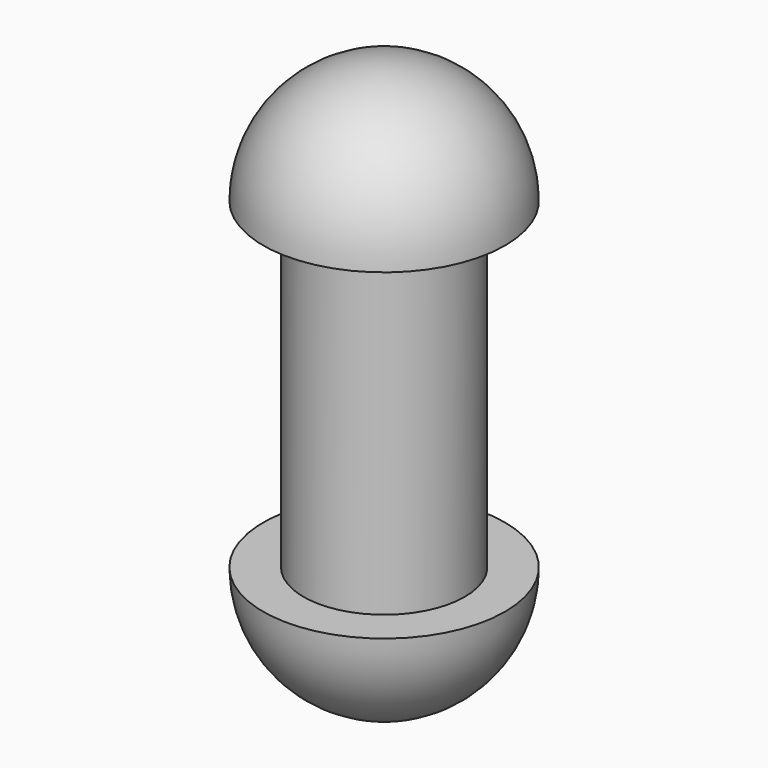
from build123d import *

# Parameters (mm, degrees)
F0_R     = 1
F1_DEPTH = 2


# Not quite as in the source:
# - a pattern or mirror of a feature is missing from the dataset's text; its kind, count and spacing are read off the source's solid


with BuildPart() as f1:
    # F0 (on Top) → F1 (new body, symmetric)
    with BuildSketch(Plane.XY):
        Circle(F0_R)
    extrude(amount=F1_DEPTH, both=True)

    # F2 (on Front) → F3 (revolve)
    with BuildSketch(Plane.XZ):
        with BuildLine():
            Line((0, 2), (1.5, 2))
            ThreePointArc((1.5, 2), (1.0606601718, 3.0606601718), (0, 3.5))
            Line((0, 3.5), (0, 2))
        make_face()
    f3 = revolve(axis=Axis((0, 0, 2.75), (0, 0, 1)))

    # F3_copies: F3 across plane
    add(f3.mirror(Plane(origin=(0, 0, 0), x_dir=(-1, 0, 0), z_dir=(0, 0, -1))))


solid = f1.part
